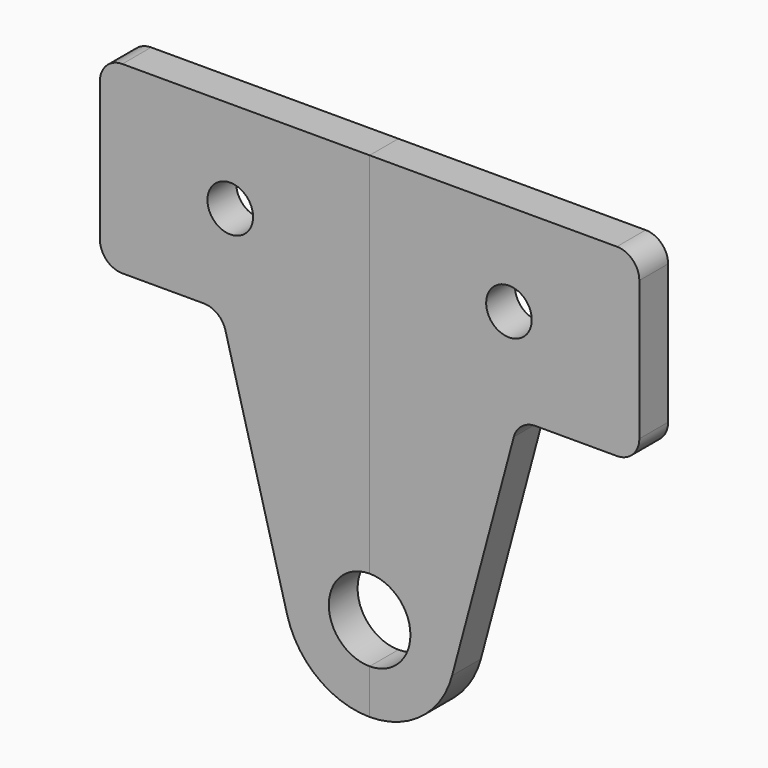
from build123d import *
from build123d import SkipClean  # not in build123d's __all__

# Parameters (mm, degrees)
F0_R     = 5.075
F1_DEPTH = 8


with BuildPart() as f1:
    # F0 (on Front) → F1 (new body)
    with BuildSketch(Plane.XZ):
        with BuildLine():
            ThreePointArc((-18.3525906995, 14.0824381431), (-11.5664671512, 3.9262865345), (0, 0))
            Line((0, 0), (0, 9.925))
            ThreePointArc((0, 9.925), (-9.075, 19), (0, 28.075))
            Line((0, 28.075), (0, 110))
            Line((0, 110), (-55, 110))
            ThreePointArc((-55, 110), (-58.5355339059, 108.5355339059), (-60, 105))
            Line((-60, 105), (-60, 74))
            ThreePointArc((-60, 74), (-58.5355339059, 70.4644660941), (-55, 69))
            Line((-55, 69), (-36.9043419892, 69))
            ThreePointArc((-36.9043419892, 69), (-33.8605348442, 67.9667667015), (-32.0747128578, 65.2940952255))
            Line((-32.0747128578, 65.2940952255), (-18.3525906995, 14.0824381431))
        make_face()
        with Locations((-31, 89.5)):
            Circle(F0_R, mode=Mode.SUBTRACT)
    extrude(amount=F1_DEPTH)

    # F2: F1 across face


with BuildPart() as f1_1:
    add(f1.part, clean=False)
    with SkipClean():  # cleaning this boolean's faces spoils the solid; the shape is the same uncleaned
        add(f1.part.mirror(Plane(origin=(0, -4, 69.0375), x_dir=(0, 1, 0), z_dir=(1, 0, 0))), clean=False)


solid = f1_1.part
